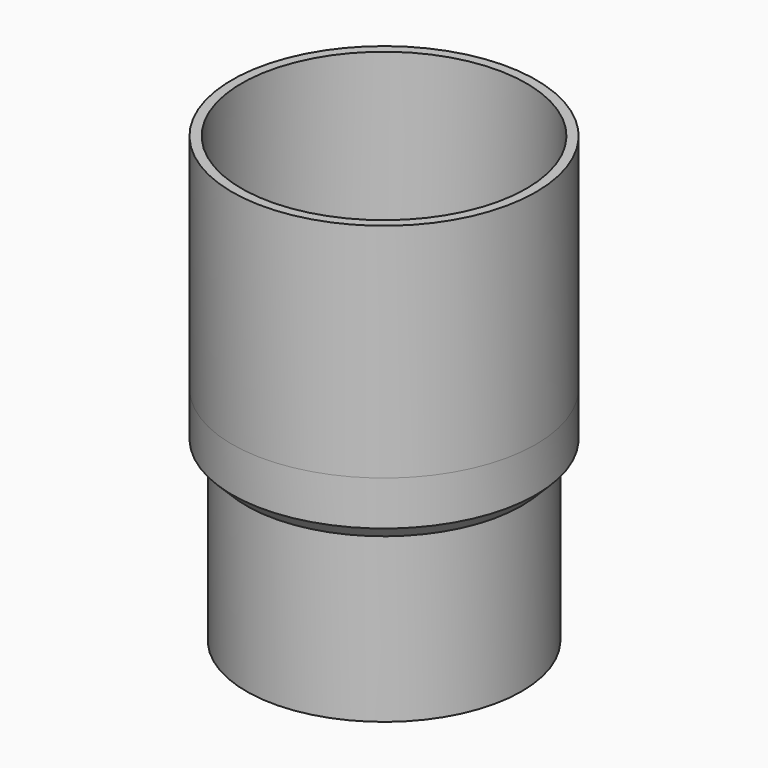
from build123d import *

# Parameters (mm, degrees)
F0_R     = 21.7
F0_R_2   = 20.2
F1_DEPTH = 35
F2_R     = 23.95
F2_R_2   = 22.45
F3_DEPTH = 35
F4_R     = 23.95
F4_R_2   = 21.7
F5_DEPTH = 10


# Not quite as in the source:
# - a fillet or chamfer that OpenCascade refuses, or shapes differently, is made with other operations: its cross-section is extruded or revolved along the edge and cut away or added


with BuildPart() as f1:
    # F0 (on Top) → F1 (new body)
    with BuildSketch(Plane.XY):
        Circle(F0_R)
        Circle(F0_R_2, mode=Mode.SUBTRACT)
    extrude(amount=F1_DEPTH)


with BuildPart() as f3:
    # F2 (on face) → F3 (new body)
    with BuildSketch(Plane.XY.offset(35)):
        Circle(F2_R)
        Circle(F2_R_2, mode=Mode.SUBTRACT)
    extrude(amount=F3_DEPTH)


with BuildPart() as f5:
    # F4 (on face) → F5 (new body)
    with BuildSketch(Plane(origin=(0, 0, 35), x_dir=(1, 0, 0), z_dir=(0, 0, -1))):
        Circle(F4_R)
        Circle(F4_R_2, mode=Mode.SUBTRACT)
    extrude(amount=F5_DEPTH)

    # F6: chamfer of 3 on 1 edges, made by hand

    # F6_s1 → F6_t2 (revolve, cut)
    with BuildSketch(Plane.XZ):
        Polygon((23.95, 28), (20.95, 25), (23.95, 25), align=None)
    revolve(axis=Axis((0, 0, 25), (0, 0, -1)), mode=Mode.SUBTRACT)


solid = Compound([f1.part, f3.part, f5.part])
